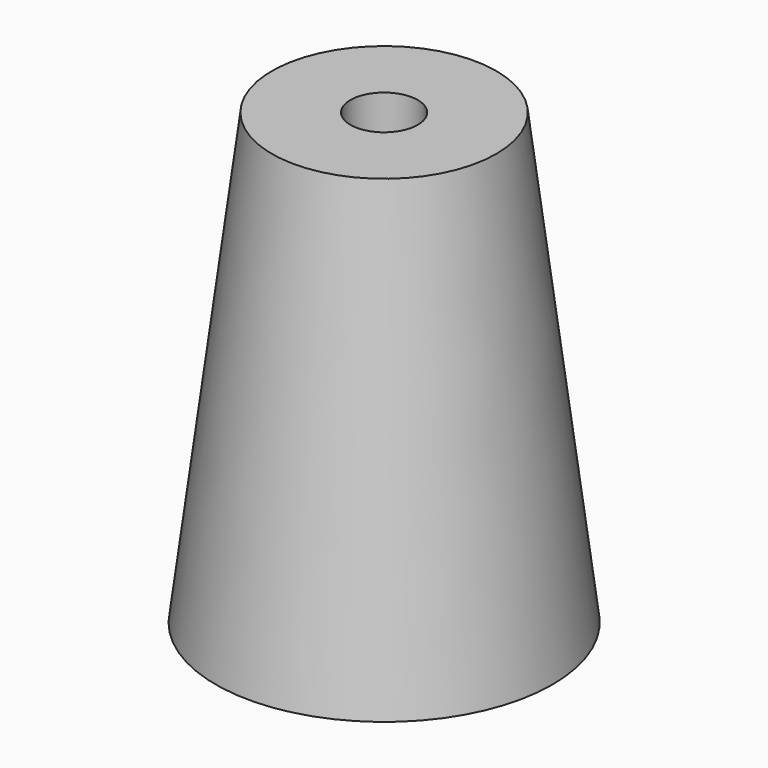
from build123d import *

# Parameters (mm, degrees)
F0_R     = 7.5
F2_R     = 5
F4_T     = -2.5
F5_R     = 1.5
F6_DEPTH = 25


with BuildPart() as f3:
    # F0 (on Top) → F3 section 0
    with BuildSketch(Plane.XY):
        Circle(F0_R)
    # F2 (on offset) → F3 section 1
    with BuildSketch(Plane.XY.offset(20)):
        Circle(F2_R)
    loft()

    # F4
    f4_openings = [f3.faces().sort_by_distance(p)[0] for p in [
        (0, 0, 0),
    ]]
    offset(amount=F4_T, openings=f4_openings, kind=Kind.INTERSECTION)

    # F5 (on face) → F6 (cut)
    with BuildSketch(Plane.XY.offset(20)):
        Circle(F5_R)
    extrude(amount=-F6_DEPTH, mode=Mode.SUBTRACT)


solid = f3.part
